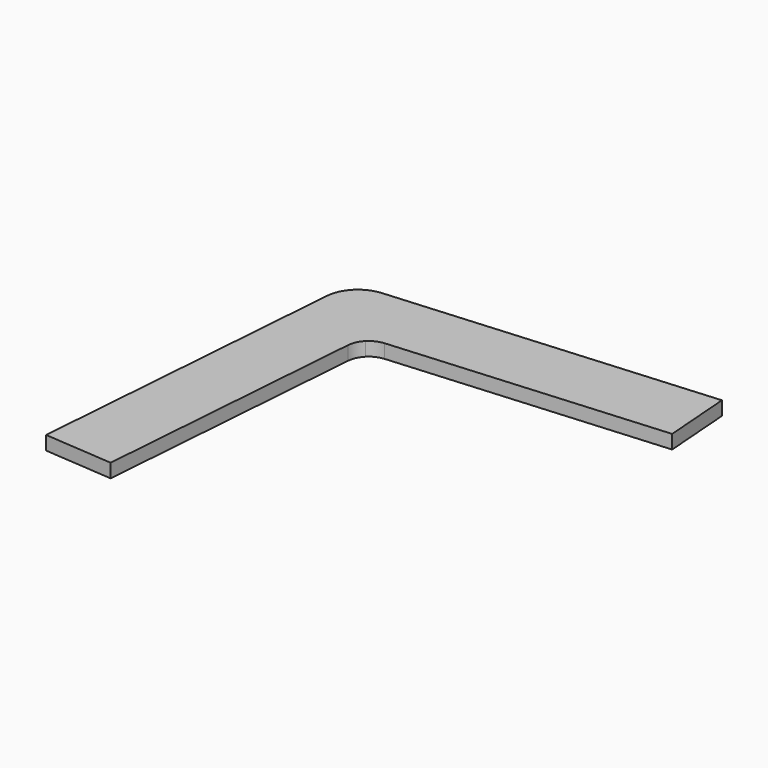
from build123d import *

# Parameters (mm, degrees)
F1_DEPTH = 5
F4_DEPTH = 5


# Not quite as in the source:
# - a feature of the source that left no trace in its solid (it failed there, or was rolled back) is left out


with BuildPart() as f1:
    # F0 (on Top) → F1 (new body)
    with BuildSketch(Plane.XY):
        with BuildLine():
            Line((67.2432569916, 68.9932702117), (-49.1140455478, 60.1726392496))
            ThreePointArc((-49.1140455478, 60.1726392496), (-53.2152003045, 59.1119075124), (-56.692252409, 56.692252409))
            Line((-56.692252409, 56.692252409), (-36.0883415168, 36.0883415168))
            Line((-36.0883415168, 36.0883415168), (-34.2875776013, 34.2875776013))
            ThreePointArc((-34.2875776013, 34.2875776013), (-31.969542865, 35.9006810036), (-29.2354396938, 36.607835495))
            Line((-29.2354396938, 36.607835495), (69.1329955604, 44.0647947641))
            Line((69.1329955604, 44.0647947641), (67.2432569916, 68.9932702117))
        make_face()
    extrude(amount=F1_DEPTH)

    # F0 (on Top) → F4 (join)
    with BuildSketch(Plane.XY):
        with BuildLine():
            Line((-36.0883415168, 36.0883415168), (-56.692252409, 56.692252409))
            ThreePointArc((-56.692252409, 56.692252409), (-59.1119075124, 53.2152003045), (-60.1726392496, 49.1140455478))
            Line((-60.1726392496, 49.1140455478), (-68.9932702117, -67.2432569916))
            Line((-68.9932702117, -67.2432569916), (-44.0647947641, -69.1329955604))
            Line((-44.0647947641, -69.1329955604), (-36.607835495, 29.2354396938))
            ThreePointArc((-36.607835495, 29.2354396938), (-35.9006810036, 31.969542865), (-34.2875776013, 34.2875776013))
            Line((-34.2875776013, 34.2875776013), (-36.0883415168, 36.0883415168))
        make_face()
    extrude(amount=F4_DEPTH)


solid = f1.part
